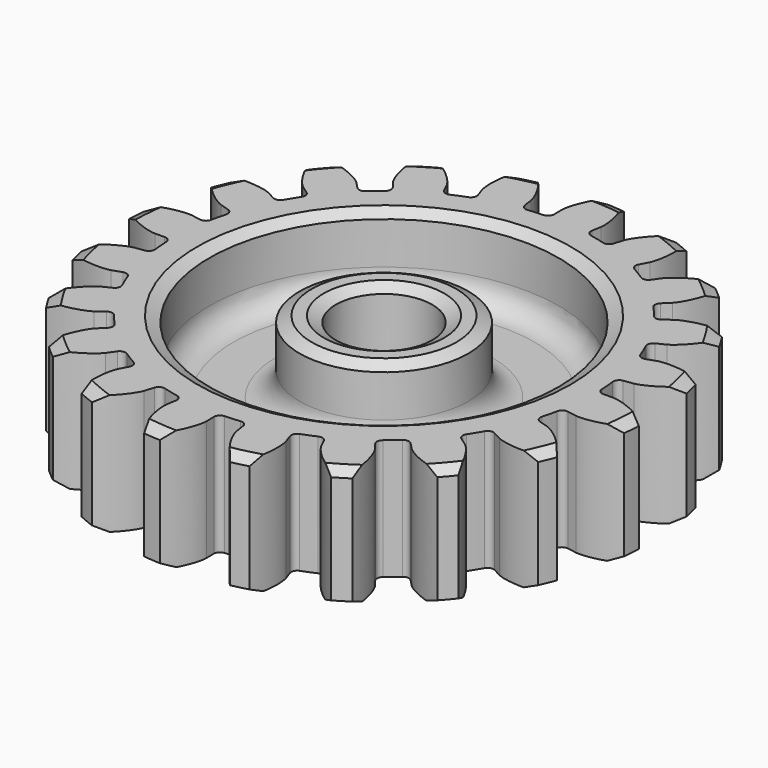
from build123d import *

# Parameters (mm, degrees)
F1_DEPTH   = 5
F2_SIZE2   = 0.25
F2_SIZE    = 0.5
F2_2_SIZE2 = 0.25
F2_2_SIZE  = 0.5
F3_COUNT   = 20
F3_ANGLE   = 342
F0_R       = 7.25
F4_DEPTH   = 5
F0_R_2     = 3.5
F0_R_3     = 2
F5_DEPTH   = 2
F6_R       = 1
F7_SIZE2   = 0.5
F7_SIZE    = 0.25
F7_2_SIZE2 = 0.5
F7_2_SIZE  = 0.25
F8_SIZE2   = 0.25
F8_SIZE    = 0.5
F8_2_SIZE2 = 0.25
F8_2_SIZE  = 0.5


# Not quite as in the source:
# - ends of sketch curves that miss each other by under 0.0002 mm in the source are joined


with BuildPart() as f1:
    # F0 (on Top) → F1 (new body)
    with BuildSketch(Plane.XY):
        with BuildLine():
            add(Edge.make_bspline(
                [(48.8696313217, -1.3602661365), (48.869788336, -1.3602917098), (48.8705730348, -1.3604198412), (48.8727686463, -1.3607893222), (48.8771818887, -1.3613871025), (48.8842786534, -1.3623098665), (48.8942409461, -1.3633827614), (48.9070677462, -1.3645730352), (48.9227689393, -1.3657449917), (48.9413458158, -1.366814071), (48.9627987651, -1.3676741178), (48.9871254822, -1.3682298678), (49.0143208068, -1.3683757318), (49.0443773151, -1.3680170526), (49.0772847213, -1.3670507092), (49.1130296098, -1.3653770863), (49.1515967141, -1.3628986532), (49.1929681087, -1.3595166442), (49.237122905, -1.355129932), (49.284037855, -1.3496420712), (49.3336872799, -1.3429573346), (49.3860423964, -1.3349737056), (49.4410732555, -1.3256010203), (49.498745062, -1.3147375318), (49.5590224811, -1.3022934422), (49.6218662303, -1.2881707563), (49.6872364173, -1.2722807293), (49.7550889597, -1.2545263946), (49.8253776298, -1.234818445), (49.8980545868, -1.2130673179), (49.9730689163, -1.1891831542), (50.0503676028, -1.1630780139), (50.1298952734, -1.1346659375), (50.2115927924, -1.1038598093), (50.2954031066, -1.0705807893), (50.3798745701, -1.0352999544), (50.4546702663, -1.0026240233), (50.5092855185, -0.9775762036), (50.5361209723, -0.9650560709), (50.5447023217, -0.9610311365)],
                knots=[0, 0, 0, 0, 0.0004772526, 0.0023852759, 0.0066791117, 0.0138360721, 0.0238549801, 0.0367361585, 0.0524806651, 0.0710868039, 0.0925563978, 0.1168879123, 0.144082354, 0.1741394035, 0.2070593458, 0.2428421037, 0.2814861216, 0.3229934797, 0.3673639947, 0.4145958591, 0.4646908312, 0.5176486068, 0.5734688008, 0.6321523041, 0.6936978179, 0.758105067, 0.8253757448, 0.8955087842, 0.9685050413, 1.0443626064, 1.1230834156, 1.2046676176, 1.2891135476, 1.3764221578, 1.4665925841, 1.5596262158, 1.6510401739, 1.7114415987, 1.7398769613, 1.7398769613, 1.7398769613, 1.7398769613], degree=3))
            ThreePointArc((50.5447023217, -0.9610311365), (50.5774269998, -0.6151500999), (50.5992126422, -0.2684081515))
            add(Edge.make_bspline(
                [(49.0072193217, 0.3879498635), (49.0073783209, 0.3879508426), (49.0081733152, 0.3879557113), (49.010399521, 0.3879744835), (49.0148515793, 0.3878774418), (49.0220050844, 0.3876764687), (49.0320126838, 0.3871792919), (49.0448678789, 0.3863480974), (49.0605594355, 0.3850487059), (49.0790747723, 0.3831988194), (49.1003985905, 0.3806932247), (49.1245124865, 0.3774346721), (49.1513965017, 0.3733269029), (49.1810264276, 0.3682691457), (49.2133769017, 0.3621665446), (49.2484201226, 0.3549234699), (49.286124905, 0.3464417842), (49.3264577501, 0.336627906), (49.3693834009, 0.3253901444), (49.4148619672, 0.3126297037), (49.4628542355, 0.2982593333), (49.5133163126, 0.2821858186), (49.5662023385, 0.2643174441), (49.6214651674, 0.2445683065), (49.6790535758, 0.2228469191), (49.7389149713, 0.1990683678), (49.8009943519, 0.1731460949), (49.8652340549, 0.1449965376), (49.9315739145, 0.1145345324), (49.9999541546, 0.0816831703), (50.07030837, 0.0463576954), (50.1425716713, 0.008482185), (50.2166755315, -0.0320203817), (50.2925474337, -0.0752294312), (50.3701202996, -0.1212089478), (50.4480327176, -0.1692696821), (50.5167961145, -0.2132428687), (50.5668199339, -0.2465266515), (50.5913662585, -0.2630904339), (50.5992126422, -0.2684081515)],
                knots=[0, 0, 0, 0, 0.0004770094, 0.0023850307, 0.0066785535, 0.0138347241, 0.023854085, 0.0367358521, 0.0524796263, 0.0710871222, 0.0925558283, 0.1168878544, 0.1440826969, 0.1741397975, 0.2070587789, 0.2428408565, 0.2814861505, 0.3229938476, 0.3673635278, 0.4145962225, 0.4646911235, 0.5176486316, 0.5734686359, 0.6321517361, 0.6936967496, 0.7581053821, 0.8253756268, 0.8955090245, 0.9685043662, 1.0443627016, 1.1230840194, 1.2046669534, 1.2891131899, 1.3764217194, 1.4665930492, 1.5596259409, 1.6510399633, 1.7114408148, 1.739876023, 1.739876023, 1.739876023, 1.739876023], degree=3))
            Line((49.0072193217, 0.3879498635), (48.6068639255, 0.3819827977))
            ThreePointArc((48.6068639255, 0.3819827977), (48.4315243184, 0.4501621192), (48.3533659584, 0.6212868354))
            ThreePointArc((48.3533659584, 0.6212868354), (48.359343504, 0.4346358787), (48.3613363217, 0.2478998635))
            ThreePointArc((48.3613363217, 0.2478998635), (48.3177251728, -0.6246212957), (48.1873264535, -1.4884449349))
            ThreePointArc((48.1873264535, -1.4884449349), (48.2912924288, -1.3316536634), (48.4751390062, -1.2917429781))
            Line((48.4751390062, -1.2917429781), (48.8696313217, -1.3602661365))
        make_face()
    extrude(amount=F1_DEPTH)

    # F2
    f2_edges = [f1.edges().sort_by_distance(p)[0] for p in [
        (50.577427, -0.61515, 5),
    ]]
    f2_side = f1.faces().sort_by_distance((49.318204, -0.516047, 5))[0]
    chamfer(f2_edges, length=F2_SIZE, length2=F2_SIZE2, reference=f2_side)

    # F2#2
    f2_2_edges = [f1.edges().sort_by_distance(p)[0] for p in [
        (50.577427, -0.61515, 0),
    ]]
    f2_2_side = f1.faces().sort_by_distance((49.318204, -0.516047, 0))[0]
    chamfer(f2_2_edges, length=F2_2_SIZE, length2=F2_2_SIZE2, reference=f2_2_side)


with BuildPart() as f3_1:
    # F3: instance of F1
    add(f1.part.rotate(Axis((39.6113363217, 0.2478998635, 0), (0, 0, 1)), 1 * F3_ANGLE / (F3_COUNT - 1)))


with BuildPart() as f3_2:
    # F3: instance of F1
    add(f1.part.rotate(Axis((39.6113363217, 0.2478998635, 0), (0, 0, 1)), 2 * F3_ANGLE / (F3_COUNT - 1)))


with BuildPart() as f3_3:
    # F3: instance of F1
    add(f1.part.rotate(Axis((39.6113363217, 0.2478998635, 0), (0, 0, 1)), 3 * F3_ANGLE / (F3_COUNT - 1)))


with BuildPart() as f3_4:
    # F3: instance of F1
    add(f1.part.rotate(Axis((39.6113363217, 0.2478998635, 0), (0, 0, 1)), 4 * F3_ANGLE / (F3_COUNT - 1)))


with BuildPart() as f3_5:
    # F3: instance of F1
    add(f1.part.rotate(Axis((39.6113363217, 0.2478998635, 0), (0, 0, 1)), 5 * F3_ANGLE / (F3_COUNT - 1)))


with BuildPart() as f3_6:
    # F3: instance of F1
    add(f1.part.rotate(Axis((39.6113363217, 0.2478998635, 0), (0, 0, 1)), 6 * F3_ANGLE / (F3_COUNT - 1)))


with BuildPart() as f3_7:
    # F3: instance of F1
    add(f1.part.rotate(Axis((39.6113363217, 0.2478998635, 0), (0, 0, 1)), 7 * F3_ANGLE / (F3_COUNT - 1)))


with BuildPart() as f3_8:
    # F3: instance of F1
    add(f1.part.rotate(Axis((39.6113363217, 0.2478998635, 0), (0, 0, 1)), 8 * F3_ANGLE / (F3_COUNT - 1)))


with BuildPart() as f3_9:
    # F3: instance of F1
    add(f1.part.rotate(Axis((39.6113363217, 0.2478998635, 0), (0, 0, 1)), 9 * F3_ANGLE / (F3_COUNT - 1)))


with BuildPart() as f3_10:
    # F3: instance of F1
    add(f1.part.rotate(Axis((39.6113363217, 0.2478998635, 0), (0, 0, 1)), 10 * F3_ANGLE / (F3_COUNT - 1)))


with BuildPart() as f3_11:
    # F3: instance of F1
    add(f1.part.rotate(Axis((39.6113363217, 0.2478998635, 0), (0, 0, 1)), 11 * F3_ANGLE / (F3_COUNT - 1)))


with BuildPart() as f3_12:
    # F3: instance of F1
    add(f1.part.rotate(Axis((39.6113363217, 0.2478998635, 0), (0, 0, 1)), 12 * F3_ANGLE / (F3_COUNT - 1)))


with BuildPart() as f3_13:
    # F3: instance of F1
    add(f1.part.rotate(Axis((39.6113363217, 0.2478998635, 0), (0, 0, 1)), 13 * F3_ANGLE / (F3_COUNT - 1)))


with BuildPart() as f3_14:
    # F3: instance of F1
    add(f1.part.rotate(Axis((39.6113363217, 0.2478998635, 0), (0, 0, 1)), 14 * F3_ANGLE / (F3_COUNT - 1)))


with BuildPart() as f3_15:
    # F3: instance of F1
    add(f1.part.rotate(Axis((39.6113363217, 0.2478998635, 0), (0, 0, 1)), 15 * F3_ANGLE / (F3_COUNT - 1)))


with BuildPart() as f3_16:
    # F3: instance of F1
    add(f1.part.rotate(Axis((39.6113363217, 0.2478998635, 0), (0, 0, 1)), 16 * F3_ANGLE / (F3_COUNT - 1)))


with BuildPart() as f3_17:
    # F3: instance of F1
    add(f1.part.rotate(Axis((39.6113363217, 0.2478998635, 0), (0, 0, 1)), 17 * F3_ANGLE / (F3_COUNT - 1)))


with BuildPart() as f3_18:
    # F3: instance of F1
    add(f1.part.rotate(Axis((39.6113363217, 0.2478998635, 0), (0, 0, 1)), 18 * F3_ANGLE / (F3_COUNT - 1)))


with BuildPart() as f3_19:
    # F3: instance of F1
    add(f1.part.rotate(Axis((39.6113363217, 0.2478998635, 0), (0, 0, 1)), 19 * F3_ANGLE / (F3_COUNT - 1)))


with BuildPart() as f1_1:
    add(f1.part)

    add(f3_1.part)  # F4 merges F3_1

    add(f3_2.part)  # F4 merges F3_2

    add(f3_3.part)  # F4 merges F3_3

    add(f3_4.part)  # F4 merges F3_4

    add(f3_5.part)  # F4 merges F3_5

    add(f3_6.part)  # F4 merges F3_6

    add(f3_7.part)  # F4 merges F3_7

    add(f3_8.part)  # F4 merges F3_8

    add(f3_9.part)  # F4 merges F3_9

    add(f3_10.part)  # F4 merges F3_10

    add(f3_11.part)  # F4 merges F3_11

    add(f3_12.part)  # F4 merges F3_12

    add(f3_13.part)  # F4 merges F3_13

    add(f3_14.part)  # F4 merges F3_14

    add(f3_15.part)  # F4 merges F3_15

    add(f3_16.part)  # F4 merges F3_16

    add(f3_17.part)  # F4 merges F3_17

    add(f3_18.part)  # F4 merges F3_18

    add(f3_19.part)  # F4 merges F3_19
    # F0 (on Top) → F4 (join)
    with BuildSketch(Plane.XY):
        with BuildLine():
            ThreePointArc((48.3533659584, 0.6212868354), (30.888309656, 0.9344170072), (48.1873264535, -1.4884449349))
            ThreePointArc((48.1873264535, -1.4884449349), (48.3177251728, -0.6246212957), (48.3613363217, 0.2478998635))
            ThreePointArc((48.3613363217, 0.2478998635), (48.359343504, 0.4346358787), (48.3533659584, 0.6212868354))
        make_face()
        with Locations((39.6113363217, 0.2478998635)):
            Circle(F0_R, mode=Mode.SUBTRACT)
    extrude(amount=F4_DEPTH)



with BuildPart() as f4:
    # F0 (on Top) → F4, piece 2 (new body)
    with BuildSketch(Plane.XY):
        with Locations((39.6113363217, 0.2478998635)):
            Circle(F0_R_2)
        with Locations((39.6113363217, 0.2478998635)):
            Circle(F0_R_3, mode=Mode.SUBTRACT)
    extrude(amount=F4_DEPTH)


with BuildPart() as f1_2:
    add(f1_1.part)

    add(f4.part)  # F5 merges F4
    # F0 (on Top) → F5 (join)
    with BuildSketch(Plane.XY):
        with Locations((39.6113363217, 0.2478998635)):
            Circle(F0_R)
        with Locations((39.6113363217, 0.2478998635)):
            Circle(F0_R_2, mode=Mode.SUBTRACT)
    extrude(amount=F5_DEPTH)

    # F6
    f6_edges = [f1_2.edges().sort_by_distance(p)[0] for p in [
        (32.361336, 0.2479, 2),
        (36.111336, 0.2479, 2),
    ]]
    fillet(f6_edges, radius=F6_R)

    # F7
    f7_edges = [f1_2.edges().sort_by_distance(p)[0] for p in [
        (32.361336, 0.2479, 5),
    ]]
    f7_side = f1_2.faces().sort_by_distance((32.361336, 0.2479, 4))[0]
    chamfer(f7_edges, length=F7_SIZE, length2=F7_SIZE2, reference=f7_side)

    # F7#2
    f7_2_edges = [f1_2.edges().sort_by_distance(p)[0] for p in [
        (37.611336, 0.2479, 5),
    ]]
    f7_2_side = f1_2.faces().sort_by_distance((37.611336, 0.2479, 2.5))[0]
    chamfer(f7_2_edges, length=F7_2_SIZE, length2=F7_2_SIZE2, reference=f7_2_side)

    # F8
    f8_edges = [f1_2.edges().sort_by_distance(p)[0] for p in [
        (36.111336, 0.2479, 5),
    ]]
    f8_side = f1_2.faces().sort_by_distance((37.012341, 0.2479, 5))[0]
    chamfer(f8_edges, length=F8_SIZE, length2=F8_SIZE2, reference=f8_side)

    # F8#2
    f8_2_edges = [f1_2.edges().sort_by_distance(p)[0] for p in [
        (37.611336, 0.2479, 0),
    ]]
    f8_2_side = f1_2.faces().sort_by_distance((37.314418, 0.2479, 0))[0]
    chamfer(f8_2_edges, length=F8_2_SIZE, length2=F8_2_SIZE2, reference=f8_2_side)


solid = f1_2.part
